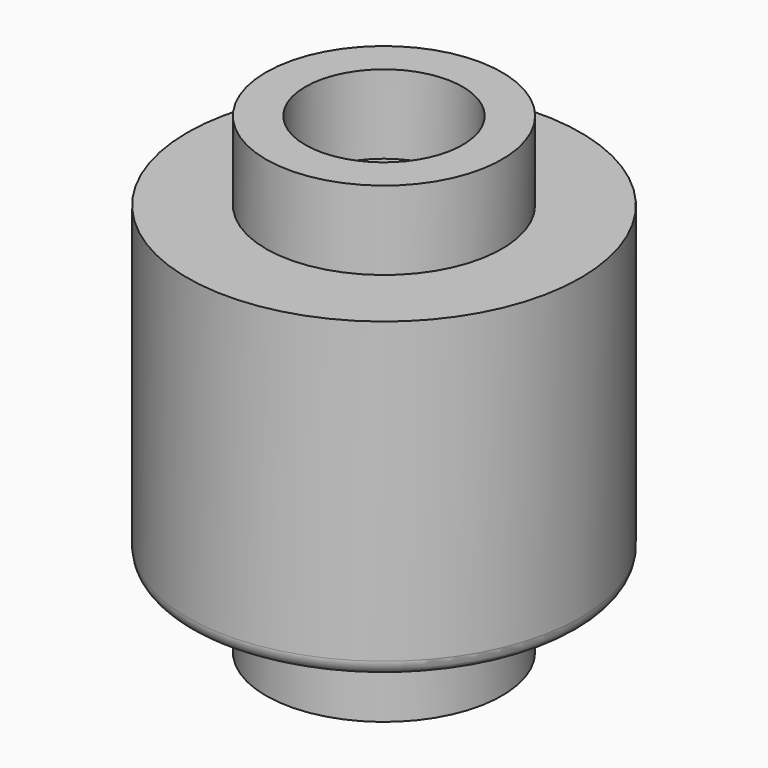
from build123d import *

# Parameters (mm, degrees)
F0_R     = 63.5
F1_DEPTH = 50.8
F2_W     = 50.8
F2_H     = 25.4
F3_DEPTH = 50.8
F5_D     = 6.35
F6_R     = 5.08
F7_R     = 5.08
F8_W     = 12.7
F8_H     = 25.4


# Not quite as in the source:
# - a pattern or mirror of a feature is missing from the dataset's text; its kind, count and spacing are read off the source's solid


with BuildPart() as f1:
    # F0 (on Top) → F1 (new body, symmetric)
    with BuildSketch(Plane.XY):
        Circle(F0_R)
    extrude(amount=F1_DEPTH, both=True)

    # F2 (on face) → F3 (cut)
    with BuildSketch(Plane.XY.offset(50.8)):
        Rectangle(F2_W, F2_H)
    extrude(amount=-F3_DEPTH, mode=Mode.SUBTRACT)

    # F5 (through all)
    with Locations(Plane(origin=(0, 0, -50.8), x_dir=(1, 0, 0), z_dir=(0, 0, -1))):
        with Locations((0, 0)):
            Hole(F5_D / 2)

    # F6
    f6_edges = [f1.edges().sort_by_distance(p)[0] for p in [
        (-63.5, 0, -50.8),
    ]]
    fillet(f6_edges, radius=F6_R)

    # F7
    f7_edges = [f1.edges().sort_by_distance(p)[0] for p in [
        (-25.4, 0, 0),
    ]]
    fillet(f7_edges, radius=F7_R)

    # F8 (on Front) → F9 (revolve)
    with BuildSketch(Plane.XZ):
        with Locations((-31.75, -63.5)):
            Rectangle(F8_W, F8_H)
    f9 = revolve(axis=Axis((0, 0, 19.3926589563), (0, 0, -1)))

    # F9_copies: F9 across plane
    add(f9.mirror(Plane.XY))


solid = f1.part
